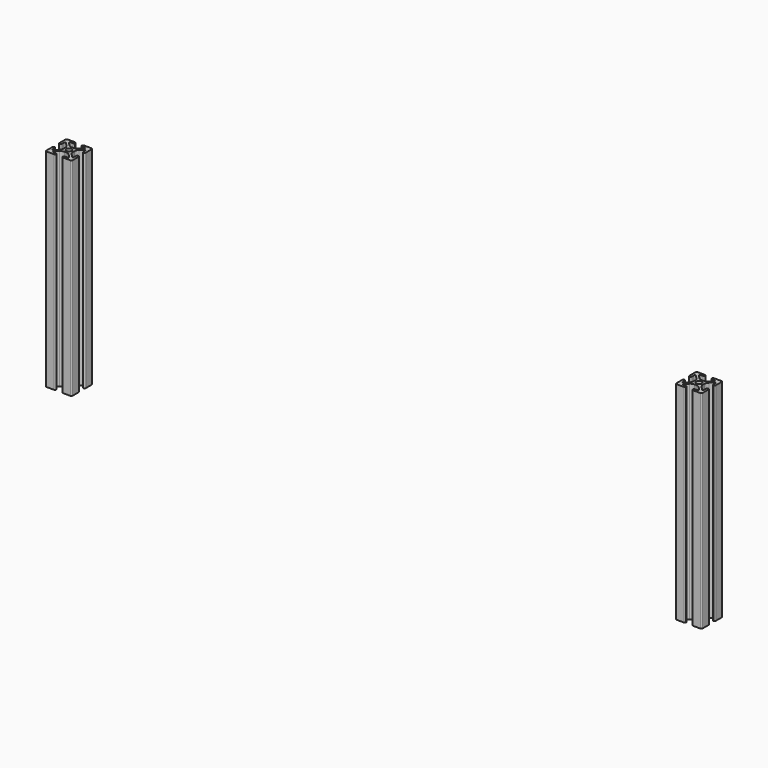
from build123d import *

# Parameters (mm, degrees)
F0_R     = 2.6035
F1_DEPTH = 200.66
F2_R     = 1.18109
F3_R     = 5.08
F4_R     = 0.762
F5_R     = 1.27


# Not quite as in the source:
# - a fillet or chamfer is up to 0.001 mm smaller than in the source, because OpenCascade refuses the exact size


with BuildPart() as f1:
    # F0 (on Top) → F1 (new body)
    with BuildSketch(Plane.XY):
        Polygon((12.7, 3.2385), (12.7, 12.7), (3.2385, 12.7), (3.2385, 10.3378), (8.7752354349, 10.3378), (2.9459354349, 4.5085), (-2.9459354349, 4.5085), (-8.7752354349, 10.3378), (-3.2385, 10.3378), (-3.2385, 12.7), (-12.7, 12.7), (-12.7, 3.2385), (-10.3378, 3.2385), (-10.3378, 8.7752354349), (-4.5085, 2.9459354349), (-4.5085, -2.9459354349), (-10.3378, -8.7752354349), (-10.3378, -3.2385), (-12.7, -3.2385), (-12.7, -12.7), (-3.2385, -12.7), (-3.2385, -10.3378), (-8.7752354349, -10.3378), (-2.9459354349, -4.5085), (2.9459354349, -4.5085), (8.7752354349, -10.3378), (3.2385, -10.3378), (3.2385, -12.7), (12.7, -12.7), (12.7, -3.2385), (10.3378, -3.2385), (10.3378, -8.7752354349), (4.5085, -2.9459354349), (4.5085, 2.9459354349), (10.3378, 8.7752354349), (10.3378, 3.2385), align=None)
        Circle(F0_R, mode=Mode.SUBTRACT)
    extrude(amount=F1_DEPTH)

    # F2 (radius 1.1811 in the source; OpenCascade refuses exactly that, so slightly less here)
    f2_edges = [f1.edges().sort_by_distance(p)[0] for p in [
        (3.2385, 12.7, 100.33),
        (3.2385, 10.3378, 100.33),
        (-3.2385, 12.7, 100.33),
        (-12.7, 3.2385, 100.33),
        (-3.2385, 10.3378, 100.33),
        (-10.3378, 3.2385, 100.33),
        (12.7, 3.2385, 100.33),
        (10.3378, 3.2385, 100.33),
        (12.7, -3.2385, 100.33),
        (10.3378, -3.2385, 100.33),
        (3.2385, -10.3378, 100.33),
        (-3.2385, -10.3378, 100.33),
        (-10.3378, -3.2385, 100.33),
        (-12.7, -3.2385, 100.33),
        (-3.2385, -12.7, 100.33),
        (3.2385, -12.7, 100.33),
    ]]
    fillet(f2_edges, radius=F2_R)

    # F3
    f3_edges = [f1.edges().sort_by_distance(p)[0] for p in [
        (2.945935, 4.5085, 100.33),
        (-2.945935, 4.5085, 100.33),
        (4.5085, -2.945935, 100.33),
        (4.5085, 2.945935, 100.33),
        (2.945935, -4.5085, 100.33),
        (-2.945935, -4.5085, 100.33),
        (-4.5085, -2.945935, 100.33),
        (-4.5085, 2.945935, 100.33),
    ]]
    fillet(f3_edges, radius=F3_R)

    # F4
    f4_edges = [f1.edges().sort_by_distance(p)[0] for p in [
        (8.775235, 10.3378, 100.33),
        (-8.775235, 10.3378, 100.33),
        (-10.3378, 8.775235, 100.33),
        (-10.3378, -8.775235, 100.33),
        (-8.775235, -10.3378, 100.33),
        (8.775235, -10.3378, 100.33),
        (10.3378, -8.775235, 100.33),
        (10.3378, 8.775235, 100.33),
    ]]
    fillet(f4_edges, radius=F4_R)

    # F5
    f5_edges = [f1.edges().sort_by_distance(p)[0] for p in [
        (-12.7, -12.7, 100.33),
        (12.7, -12.7, 100.33),
        (12.7, 12.7, 100.33),
        (-12.7, 12.7, 100.33),
    ]]
    fillet(f5_edges, radius=F5_R)


with BuildPart() as f6_1:
    # F6: copy of F1
    add(f1.part.moved(Location((609.6, 0, 0))))


solid = Compound([f1.part, f6_1.part])
